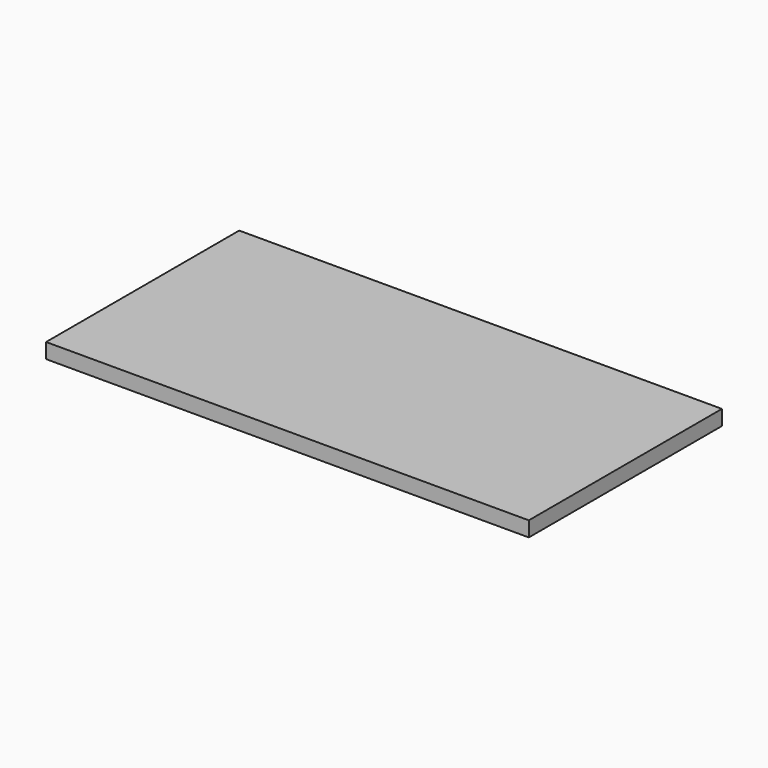
from build123d import *

# Parameters (mm, degrees)
F1_W     = 203.2
F1_H     = 101.6
F2_DEPTH = 6.35


# Not quite as in the source:
# - a length typed as a fraction of an inch, garbled in the dataset ("3 / 203.2 mm" for 3/8 in), is restored


with BuildPart() as f2:
    # F1 (on Top) → F2 (new body)
    with BuildSketch(Plane.XY):
        with Locations((101.6, 50.8)):
            Rectangle(F1_W, F1_H)
    extrude(amount=F2_DEPTH)


solid = f2.part
